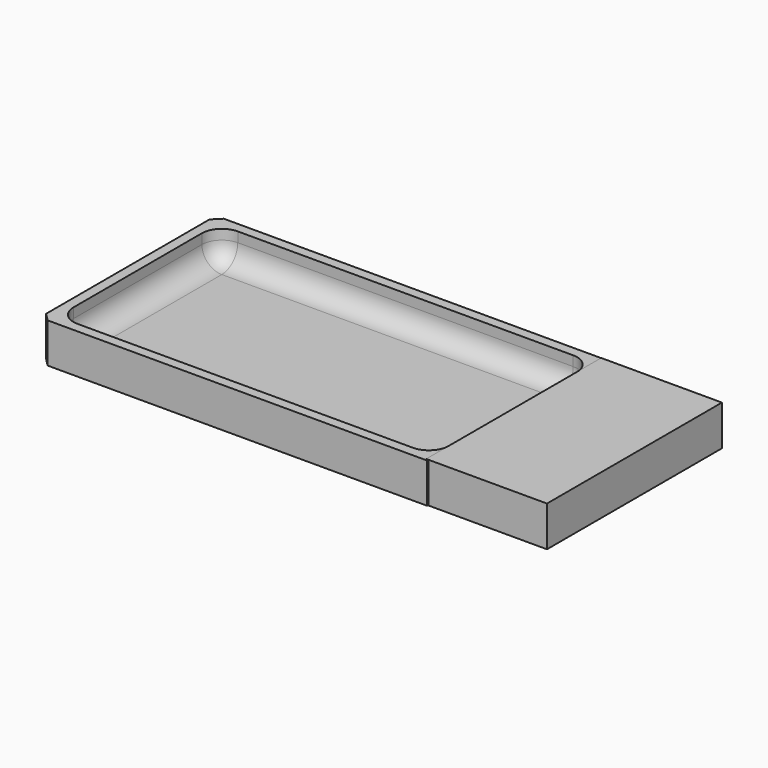
from build123d import *

# Parameters (mm, degrees)
F0_W         = 99.2175191641
F0_H         = 55.2872437984
F1_DEPTH     = 10
F2_T         = -2.5
F3_R         = 5
F4_T1_DEPTH  = 2.5
F4_S5_W      = 5
F4_S5_H      = 5
F4_T6_DEPTH  = 5
F4_S11_W     = 5
F4_S11_H     = 5
F4_T12_DEPTH = 5
F4_S17_W     = 5
F4_S17_H     = 5
F4_T18_DEPTH = 5
F4_S23_W     = 5
F4_S23_H     = 5
F4_T24_DEPTH = 5
F5_SIZE      = 2
F6_W         = 2.7456413954
F6_H         = 3.2448493876
F6_W_2       = 2.9952451587
F6_H_2       = 3.1200476224
F7_DEPTH     = 58.81103
F8_W         = 30.3268581629
F8_H         = 54.9128409475
F9_DEPTH     = 10.11623


# Not quite as in the source:
# - a fillet or chamfer that OpenCascade refuses, or shapes differently, is made with other operations: its cross-section is extruded or revolved along the edge and cut away or added
# - a feature names something its author has since deleted; it is built from what else it names


with BuildPart() as f1:
    # F0 (on Top) → F1 (new body)
    with BuildSketch(Plane.XY):
        with Locations((6.4272992313, 3.9312606677)):
            Rectangle(F0_W, F0_H)
    extrude(amount=F1_DEPTH)

    # F2
    f2_openings = [f1.faces().sort_by_distance(p)[0] for p in [
        (6.427299, 3.931261, 10),
    ]]
    offset(amount=F2_T, openings=f2_openings)

    # F3
    f3_edges = [f1.edges().sort_by_distance(p)[0] for p in [
        (6.427299, 29.074883, 2.5),
        (-40.68146, 3.931261, 2.5),
        (53.536059, 3.931261, 2.5),
        (6.427299, -21.212361, 2.5),
    ]]
    fillet(f3_edges, radius=F3_R)

    # F4: fillet of radius 5 on 4 edges, made by hand

    # F4_s2 → F4_t1 (join)
    with BuildSketch(Plane.XY.offset(7.5)):
        with BuildLine():
            ThreePointArc((-35.6814603508, 29.0748825669), (-39.2169942567, 27.6104164729), (-40.6814603508, 24.0748825669))
            Line((-40.6814603508, 24.0748825669), (-40.6814603508, 29.0748825669))
            Line((-40.6814603508, 29.0748825669), (-35.6814603508, 29.0748825669))
        make_face()
        with BuildLine():
            ThreePointArc((-40.6814603508, -16.2123612314), (-39.2169942567, -19.7478951374), (-35.6814603508, -21.2123612314))
            Line((-35.6814603508, -21.2123612314), (-40.6814603508, -21.2123612314))
            Line((-40.6814603508, -21.2123612314), (-40.6814603508, -16.2123612314))
        make_face()
        with BuildLine():
            ThreePointArc((53.5360588133, -16.2123612314), (52.0715927193, -19.7478951374), (48.5360588133, -21.2123612314))
            Line((48.5360588133, -21.2123612314), (53.5360588133, -21.2123612314))
            Line((53.5360588133, -21.2123612314), (53.5360588133, -16.2123612314))
        make_face()
        with BuildLine():
            ThreePointArc((48.5360588133, 29.0748825669), (52.0715927193, 27.6104164729), (53.5360588133, 24.0748825669))
            Line((53.5360588133, 24.0748825669), (53.5360588133, 29.0748825669))
            Line((53.5360588133, 29.0748825669), (48.5360588133, 29.0748825669))
        make_face()
    extrude(amount=F4_T1_DEPTH)


with BuildPart() as f4_tool4:
    # F4_s5 → F4_t6 (new body)
    with BuildSketch(Plane.XZ.offset(-24.0748825669)):
        with Locations((51.0360588133, 5)):
            Rectangle(F4_S5_W, F4_S5_H)
    extrude(amount=-F4_T6_DEPTH)

    # F4_s7 → F4_t8 (revolve, cut)
    with BuildSketch(Plane(origin=(48.5360588133, 24.0748825669, 7.5), x_dir=(-0.7071067812, 0, 0.7071067812), z_dir=(-0.7071067812, 0, -0.7071067812))):
        with BuildLine():
            ThreePointArc((0, -5), (5, 0), (0, 5))
            Line((0, 5), (0, -5))
        make_face()
    revolve(axis=Axis((48.5360588133, 24.0748825669, 7.5), (0, 1, 0)), mode=Mode.SUBTRACT)


with BuildPart() as f1_1:
    add(f1.part)

    # F4_t3: union F4_tool4
    add(f4_tool4.part)


with BuildPart() as f4_tool10:
    # F4_s11 → F4_t12 (new body)
    with BuildSketch(Plane.YZ.offset(48.5360588133)):
        with Locations((-18.7123612314, 5)):
            Rectangle(F4_S11_W, F4_S11_H)
    extrude(amount=F4_T12_DEPTH)

    # F4_s13 → F4_t14 (revolve, cut)
    with BuildSketch(Plane(origin=(48.5360588133, -16.2123612314, 7.5), x_dir=(0, 0.7071067812, 0.7071067812), z_dir=(0, 0.7071067812, -0.7071067812))):
        with BuildLine():
            ThreePointArc((0, -5), (5, 0), (0, 5))
            Line((0, 5), (0, -5))
        make_face()
    revolve(axis=Axis((48.5360588133, -16.2123612314, 7.5), (1, 0, 0)), mode=Mode.SUBTRACT)


with BuildPart() as f1_2:
    add(f1_1.part)

    # F4_t9: union F4_tool10
    add(f4_tool10.part)


with BuildPart() as f4_tool16:
    # F4_s17 → F4_t18 (new body)
    with BuildSketch(Plane.YZ.offset(-35.6814603508)):
        with Locations((-18.7123612314, 5)):
            Rectangle(F4_S17_W, F4_S17_H)
    extrude(amount=-F4_T18_DEPTH)

    # F4_s19 → F4_t20 (revolve, cut)
    with BuildSketch(Plane(origin=(-35.6814603508, -16.2123612314, 7.5), x_dir=(0, 0.7071067812, 0.7071067812), z_dir=(0, -0.7071067812, 0.7071067812))):
        with BuildLine():
            ThreePointArc((0, -5), (5, 0), (0, 5))
            Line((0, 5), (0, -5))
        make_face()
    revolve(axis=Axis((-35.6814603508, -16.2123612314, 7.5), (-1, 0, 0)), mode=Mode.SUBTRACT)


with BuildPart() as f1_3:
    add(f1_2.part)

    # F4_t15: union F4_tool16
    add(f4_tool16.part)


with BuildPart() as f4_tool22:
    # F4_s23 → F4_t24 (new body)
    with BuildSketch(Plane.XZ.offset(-24.0748825669)):
        with Locations((-38.1814603508, 5)):
            Rectangle(F4_S23_W, F4_S23_H)
    extrude(amount=-F4_T24_DEPTH)

    # F4_s25 → F4_t26 (revolve, cut)
    with BuildSketch(Plane(origin=(-35.6814603508, 24.0748825669, 7.5), x_dir=(0.7071067812, 0, 0.7071067812), z_dir=(-0.7071067812, 0, 0.7071067812))):
        with BuildLine():
            ThreePointArc((0, -5), (5, 0), (0, 5))
            Line((0, 5), (0, -5))
        make_face()
    revolve(axis=Axis((-35.6814603508, 24.0748825669, 7.5), (0, 1, 0)), mode=Mode.SUBTRACT)


with BuildPart() as f1_4:
    add(f1_3.part)

    # F4_t21: union F4_tool22
    add(f4_tool22.part)

    # F5
    f5_edges = [f1_4.edges().sort_by_distance(p)[0] for p in [
        (56.036059, -23.712361, 5),
        (56.036059, 31.574883, 5),
        (-43.18146, -23.712361, 5),
        (-43.18146, 31.574883, 5),
    ]]
    chamfer(f5_edges, length=F5_SIZE)

    # F6 (on Right) → F7 (cut, symmetric)
    with BuildSketch(Plane.YZ):
        with Locations((-13.6034078896, -0.1248018816)):
            Rectangle(F6_W, F6_H)
        with Locations((19.7187010199, -0.3120047622)):
            Rectangle(F6_W_2, F6_H_2)
    extrude(amount=F7_DEPTH, both=True, mode=Mode.SUBTRACT)

    # F8 (on Top) → F9 (join)
    with BuildSketch(Plane.XY):
        with Locations((68.8282549381, 3.9936611429)):
            Rectangle(F8_W, F8_H)
    extrude(amount=F9_DEPTH)


solid = f1_4.part
